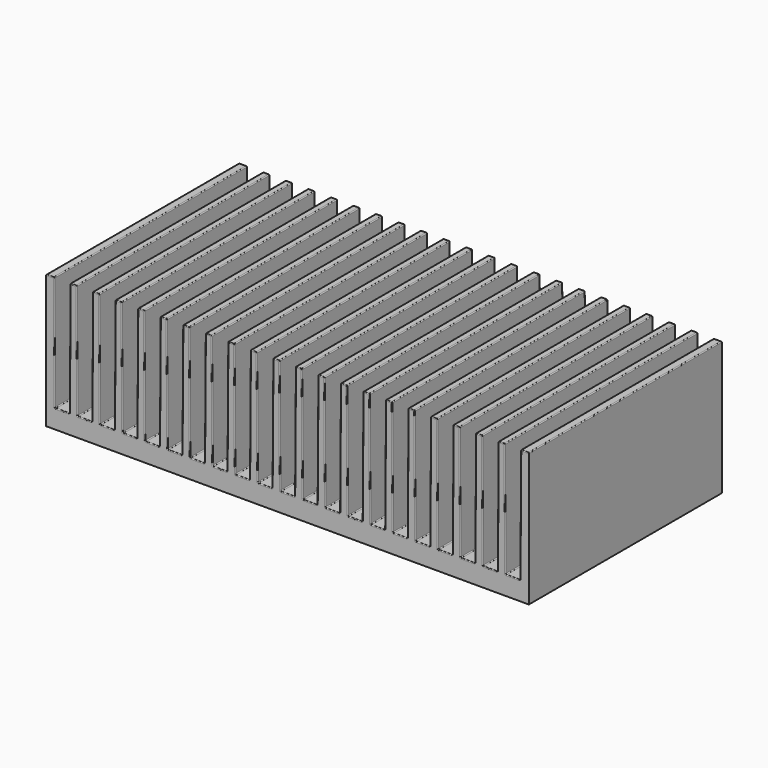
from build123d import *

# Parameters (mm, degrees)
F1_DEPTH = 150
F2_F1_R  = 0.5
F2_F2_R  = 0.5


with BuildPart() as f1:
    # F0 (on Front) → F1 (new body)
    with BuildSketch(Plane.XZ):
        Polygon((4.5, 0), (0, 0), (-4.5, 0), (-5, 71.3), (-9, 71.3), (-10, 71.3), (-10, -11.7), (290, -11.7), (290, 71.3), (285, 71.3), (284.5, 0), (280, 0), (275.5, 0), (275, 71.3), (271, 71.3), (270.5, 0), (266, 0), (261.5, 0), (261, 71.3), (257, 71.3), (256.5, 0), (252, 0), (247.5, 0), (247, 71.3), (243, 71.3), (242.5, 0), (238, 0), (233.5, 0), (233, 71.3), (229, 71.3), (228.5, 0), (224, 0), (219.5, 0), (219, 71.3), (215, 71.3), (214.5, 0), (210, 0), (205.5, 0), (205, 71.3), (201, 71.3), (200.5, 0), (196, 0), (191.5, 0), (191, 71.3), (187, 71.3), (186.5, 0), (182, 0), (177.5, 0), (177, 71.3), (173, 71.3), (172.5, 0), (168, 0), (163.5, 0), (163, 71.3), (159, 71.3), (158.5, 0), (154, 0), (149.5, 0), (149, 71.3), (145, 71.3), (144.5, 0), (140, 0), (135.5, 0), (135, 71.3), (131, 71.3), (130.5, 0), (126, 0), (121.5, 0), (121, 71.3), (117, 71.3), (116.5, 0), (112, 0), (107.5, 0), (107, 71.3), (103, 71.3), (102.5, 0), (98, 0), (93.5, 0), (93, 71.3), (89, 71.3), (88.5, 0), (84, 0), (79.5, 0), (79, 71.3), (75, 71.3), (74.5, 0), (70, 0), (65.5, 0), (65, 71.3), (61, 71.3), (60.5, 0), (56, 0), (51.5, 0), (51, 71.3), (47, 71.3), (46.5, 0), (42, 0), (37.5, 0), (37, 71.3), (33, 71.3), (32.5, 0), (28, 0), (23.5, 0), (23, 71.3), (19, 71.3), (18.5, 0), (14, 0), (9.5, 0), (9, 71.3), (5, 71.3), align=None)
    extrude(amount=F1_DEPTH)

    # F2: fillet of radius 0.5 on 172 edges, made by hand

    # F2_f1
    f2_f1_edges = [f1.edges().sort_by_distance(p)[0] for p in [
        (284.5, -75, 0),
        (275.5, -75, 0),
        (270.5, -75, 0),
        (261.5, -75, 0),
        (256.5, -75, 0),
        (247.5, -75, 0),
        (242.5, -75, 0),
        (233.5, -75, 0),
        (228.5, -75, 0),
        (219.5, -75, 0),
        (214.5, -75, 0),
        (205.5, -75, 0),
        (200.5, -75, 0),
        (191.5, -75, 0),
        (186.5, -75, 0),
        (177.5, -75, 0),
        (172.5, -75, 0),
        (163.5, -75, 0),
        (158.5, -75, 0),
        (149.5, -75, 0),
        (144.5, -75, 0),
        (135.5, -75, 0),
        (130.5, -75, 0),
        (121.5, -75, 0),
        (116.5, -75, 0),
        (107.5, -75, 0),
        (102.5, -75, 0),
        (93.5, -75, 0),
        (88.5, -75, 0),
        (79.5, -75, 0),
        (74.5, -75, 0),
        (65.5, -75, 0),
        (60.5, -75, 0),
        (51.5, -75, 0),
        (46.5, -75, 0),
        (37.5, -75, 0),
        (32.5, -75, 0),
        (23.5, -75, 0),
        (18.5, -75, 0),
        (9.5, -75, 0),
        (4.5, -75, 0),
        (-4.5, -75, 0),
    ]]
    fillet(f2_f1_edges, radius=F2_F1_R)

    # F2_f2
    f2_f2_edges = [f1.edges().sort_by_distance(p)[0] for p in [
        (-5, -75, 71.3),
        (-7.5, -150, 71.3),
        (-10, -75, 71.3),
        (-7.5, 0, 71.3),
        (9, -75, 71.3),
        (5, -75, 71.3),
        (7, 0, 71.3),
        (7, -150, 71.3),
        (23, -75, 71.3),
        (19, -75, 71.3),
        (21, 0, 71.3),
        (21, -150, 71.3),
        (37, -75, 71.3),
        (33, -75, 71.3),
        (35, 0, 71.3),
        (35, -150, 71.3),
        (51, -75, 71.3),
        (47, -75, 71.3),
        (49, 0, 71.3),
        (49, -150, 71.3),
        (65, -75, 71.3),
        (61, -75, 71.3),
        (63, 0, 71.3),
        (63, -150, 71.3),
        (79, -75, 71.3),
        (75, -75, 71.3),
        (77, 0, 71.3),
        (77, -150, 71.3),
        (93, -75, 71.3),
        (89, -75, 71.3),
        (91, 0, 71.3),
        (91, -150, 71.3),
        (107, -75, 71.3),
        (103, -75, 71.3),
        (105, 0, 71.3),
        (105, -150, 71.3),
        (121, -75, 71.3),
        (117, -75, 71.3),
        (119, 0, 71.3),
        (119, -150, 71.3),
        (135, -75, 71.3),
        (131, -75, 71.3),
        (133, 0, 71.3),
        (133, -150, 71.3),
        (149, -75, 71.3),
        (145, -75, 71.3),
        (147, 0, 71.3),
        (147, -150, 71.3),
        (163, -75, 71.3),
        (159, -75, 71.3),
        (161, 0, 71.3),
        (161, -150, 71.3),
        (177, -75, 71.3),
        (173, -75, 71.3),
        (175, 0, 71.3),
        (175, -150, 71.3),
        (191, -75, 71.3),
        (187, -75, 71.3),
        (189, 0, 71.3),
        (189, -150, 71.3),
        (205, -75, 71.3),
        (201, -75, 71.3),
        (203, 0, 71.3),
        (203, -150, 71.3),
        (219, -75, 71.3),
        (215, -75, 71.3),
        (217, 0, 71.3),
        (217, -150, 71.3),
        (233, -75, 71.3),
        (229, -75, 71.3),
        (231, 0, 71.3),
        (231, -150, 71.3),
        (247, -75, 71.3),
        (243, -75, 71.3),
        (245, 0, 71.3),
        (245, -150, 71.3),
        (261, -75, 71.3),
        (257, -75, 71.3),
        (259, 0, 71.3),
        (259, -150, 71.3),
        (275, -75, 71.3),
        (271, -75, 71.3),
        (273, 0, 71.3),
        (273, -150, 71.3),
        (290, -75, 71.3),
        (285, -75, 71.3),
        (287.5, 0, 71.3),
        (287.5, -150, 71.3),
        (280, -150, 0),
        (280, 0, 0),
        (266, -150, 0),
        (266, 0, 0),
        (252, -150, 0),
        (252, 0, 0),
        (238, -150, 0),
        (238, 0, 0),
        (224, -150, 0),
        (224, 0, 0),
        (210, -150, 0),
        (210, 0, 0),
        (196, -150, 0),
        (196, 0, 0),
        (182, -150, 0),
        (182, 0, 0),
        (168, -150, 0),
        (168, 0, 0),
        (154, -150, 0),
        (154, 0, 0),
        (140, -150, 0),
        (140, 0, 0),
        (126, -150, 0),
        (126, 0, 0),
        (112, -150, 0),
        (112, 0, 0),
        (98, -150, 0),
        (98, 0, 0),
        (84, -150, 0),
        (84, 0, 0),
        (70, -150, 0),
        (70, 0, 0),
        (56, -150, 0),
        (56, 0, 0),
        (42, -150, 0),
        (42, 0, 0),
        (28, -150, 0),
        (28, 0, 0),
        (14, -150, 0),
        (14, 0, 0),
        (0, -150, 0),
        (0, 0, 0),
        (4.3558055892, 0, 0.1452091373),
        (-4.3558055892, 0, 0.1452091373),
        (-4.3558055892, -150, 0.1452091373),
        (4.3558055892, -150, 0.1452091373),
        (18.3558055892, 0, 0.1452091373),
        (9.6441944108, 0, 0.1452091373),
        (9.6441944108, -150, 0.1452091373),
        (18.3558055892, -150, 0.1452091373),
        (32.3558055892, 0, 0.1452091373),
        (23.6441944108, 0, 0.1452091373),
        (23.6441944108, -150, 0.1452091373),
        (32.3558055892, -150, 0.1452091373),
        (46.3558055892, 0, 0.1452091373),
        (37.6441944108, 0, 0.1452091373),
        (37.6441944108, -150, 0.1452091373),
        (46.3558055892, -150, 0.1452091373),
        (60.3558055892, 0, 0.1452091373),
        (51.6441944108, 0, 0.1452091373),
        (51.6441944108, -150, 0.1452091373),
        (60.3558055892, -150, 0.1452091373),
        (74.3558055892, 0, 0.1452091373),
        (65.6441944108, 0, 0.1452091373),
        (65.6441944108, -150, 0.1452091373),
        (74.3558055892, -150, 0.1452091373),
        (88.3558055892, 0, 0.1452091373),
        (79.6441944108, 0, 0.1452091373),
        (79.6441944108, -150, 0.1452091373),
        (88.3558055892, -150, 0.1452091373),
        (102.3558055892, 0, 0.1452091373),
        (93.6441944108, 0, 0.1452091373),
        (93.6441944108, -150, 0.1452091373),
        (102.3558055892, -150, 0.1452091373),
        (116.3558055892, 0, 0.1452091373),
        (107.6441944108, 0, 0.1452091373),
        (107.6441944108, -150, 0.1452091373),
        (116.3558055892, -150, 0.1452091373),
        (130.3558055892, 0, 0.1452091373),
        (121.6441944108, 0, 0.1452091373),
        (121.6441944108, -150, 0.1452091373),
        (130.3558055892, -150, 0.1452091373),
        (144.3558055892, 0, 0.1452091373),
        (135.6441944108, 0, 0.1452091373),
        (135.6441944108, -150, 0.1452091373),
        (144.3558055892, -150, 0.1452091373),
        (158.3558055892, 0, 0.1452091373),
        (149.6441944108, 0, 0.1452091373),
        (149.6441944108, -150, 0.1452091373),
        (158.3558055892, -150, 0.1452091373),
        (172.3558055892, 0, 0.1452091373),
        (163.6441944108, 0, 0.1452091373),
        (163.6441944108, -150, 0.1452091373),
        (172.3558055892, -150, 0.1452091373),
        (186.3558055892, 0, 0.1452091373),
        (177.6441944108, 0, 0.1452091373),
        (177.6441944108, -150, 0.1452091373),
        (186.3558055892, -150, 0.1452091373),
        (200.3558055892, 0, 0.1452091373),
        (191.6441944108, 0, 0.1452091373),
        (191.6441944108, -150, 0.1452091373),
        (200.3558055892, -150, 0.1452091373),
        (214.3558055892, 0, 0.1452091373),
        (205.6441944108, 0, 0.1452091373),
        (205.6441944108, -150, 0.1452091373),
        (214.3558055892, -150, 0.1452091373),
        (228.3558055892, 0, 0.1452091373),
        (219.6441944108, 0, 0.1452091373),
        (219.6441944108, -150, 0.1452091373),
        (228.3558055892, -150, 0.1452091373),
        (242.3558055892, 0, 0.1452091373),
        (233.6441944108, 0, 0.1452091373),
        (233.6441944108, -150, 0.1452091373),
        (242.3558055892, -150, 0.1452091373),
        (256.3558055892, 0, 0.1452091373),
        (247.6441944108, 0, 0.1452091373),
        (247.6441944108, -150, 0.1452091373),
        (256.3558055892, -150, 0.1452091373),
        (270.3558055892, 0, 0.1452091373),
        (261.6441944108, 0, 0.1452091373),
        (261.6441944108, -150, 0.1452091373),
        (270.3558055892, -150, 0.1452091373),
        (284.3558055892, 0, 0.1452091373),
        (275.6441944108, 0, 0.1452091373),
        (275.6441944108, -150, 0.1452091373),
        (284.3558055892, -150, 0.1452091373),
    ]]
    fillet(f2_f2_edges, radius=F2_F2_R)


solid = f1.part
